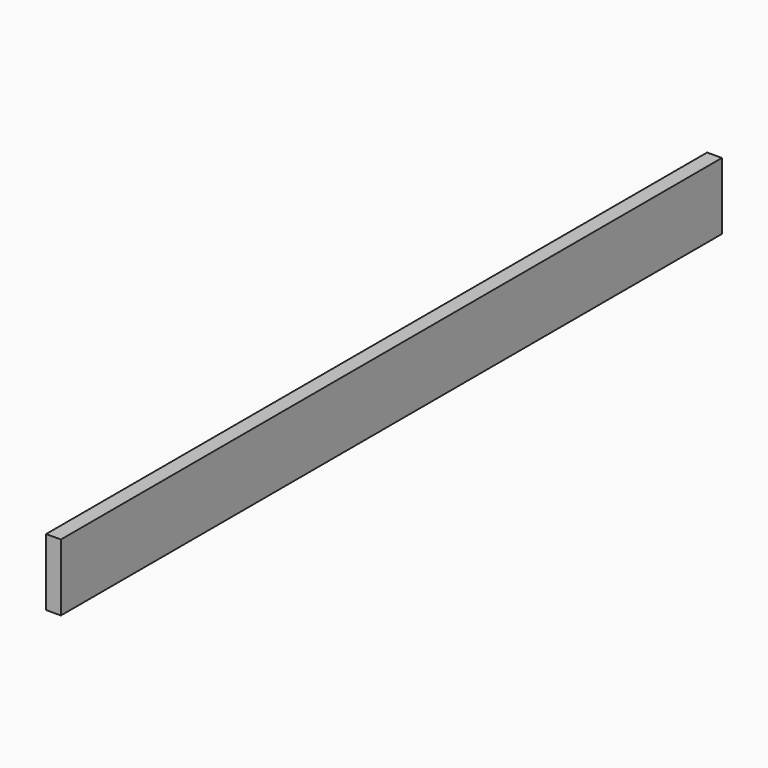
from build123d import *

# Parameters (mm, degrees)
F1_W     = 21
F1_H     = 95
F2_DEPTH = 1173


with BuildPart() as f2:
    # F1 (on Front) → F2 (new body)
    with BuildSketch(Plane.XZ):
        with Locations((10.5, 47.5)):
            Rectangle(F1_W, F1_H)
    extrude(amount=F2_DEPTH)


solid = f2.part
